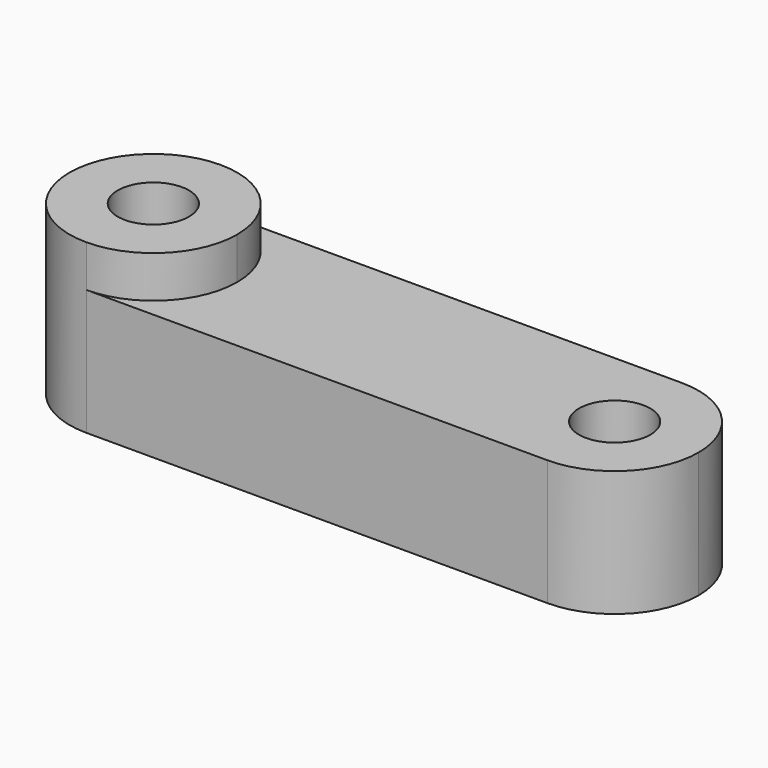
from build123d import *

# Parameters (mm, degrees)
F0_W     = 30
F0_H     = 8
F0_R     = 1.7
F1_DEPTH = 6
F2_W     = 8
F2_H     = 8
F2_R     = 1.7
F3_DEPTH = 2
F4_R     = 3.99999


# Not quite as in the source:
# - a fillet or chamfer is up to 0.001 mm smaller than in the source, because OpenCascade refuses the exact size


with BuildPart() as f1:
    # F0 (on Top) → F1 (new body)
    with BuildSketch(Plane.XY):
        Rectangle(F0_W, F0_H)
        with Locations((-11, 0)):
            Circle(F0_R, mode=Mode.SUBTRACT)
        with Locations((11, 0)):
            Circle(F0_R, mode=Mode.SUBTRACT)
    extrude(amount=F1_DEPTH)

    # F2 (on face) → F3 (join)
    with BuildSketch(Plane.XY.offset(6)):
        with Locations((-11, 0)):
            Rectangle(F2_W, F2_H)
        with Locations((-11, 0)):
            Circle(F2_R, mode=Mode.SUBTRACT)
    extrude(amount=F3_DEPTH)

    # F4 (radius 4 in the source; OpenCascade refuses exactly that, so slightly less here)
    f4_edges = [f1.edges().sort_by_distance(p)[0] for p in [
        (-15, 4, 4),
        (-15, -4, 4),
        (15, 4, 3),
        (15, -4, 3),
        (-7, -4, 7),
        (-7, 4, 7),
    ]]
    fillet(f4_edges, radius=F4_R)


solid = f1.part
